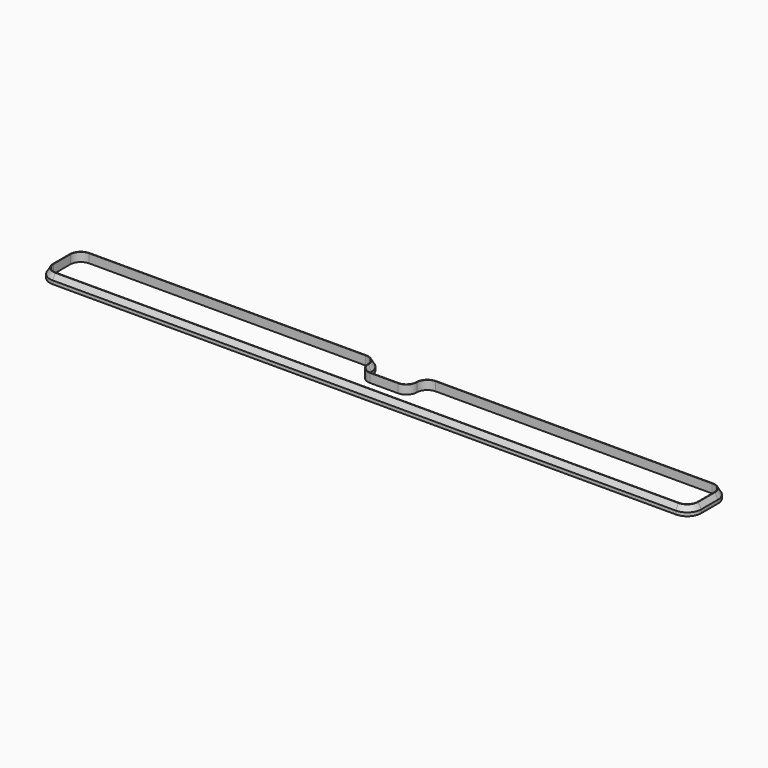
from build123d import *

# Parameters (mm, degrees)
F1_DEPTH = 8.5
F3_DEPTH = 8.501
F5_DEPTH = 8.501
F6_R     = 13.49999
F7_SIZE2 = 5.1961524227
F7_SIZE  = 3


# Not quite as in the source:
# - a fillet or chamfer is up to 0.001 mm smaller than in the source, because OpenCascade refuses the exact size


with BuildPart() as f1:
    # F0 (on Top) → F1 (new body)
    with BuildSketch(Plane.XY):
        with BuildLine():
            Line((-298.5, -23.5), (298.5, -23.5))
            ThreePointArc((298.5, -23.5), (308.045941546, -19.545941546), (312, -10))
            Line((312, -10), (312, 10))
            ThreePointArc((312, 10), (308.045941546, 19.545941546), (298.5, 23.5))
            Line((298.5, 23.5), (-298.5, 23.5))
            ThreePointArc((-298.5, 23.5), (-308.045941546, 19.545941546), (-312, 10))
            Line((-312, 10), (-312, -10))
            ThreePointArc((-312, -10), (-308.045941546, -19.545941546), (-298.5, -23.5))
        make_face()
    extrude(amount=F1_DEPTH)

    # F2 (on face) → F3 (cut, through all)
    with BuildSketch(Plane.XY.offset(8.5)):
        with BuildLine():
            Line((-13.5, 3.5), (13.5, 3.5))
            ThreePointArc((13.5, 3.5), (18.0961940777, 5.4038059223), (20, 10))
            Line((20, 10), (20, 23.5))
            Line((20, 23.5), (-20, 23.5))
            Line((-20, 23.5), (-20, 10))
            ThreePointArc((-20, 10), (-18.0961940777, 5.4038059223), (-13.5, 3.5))
        make_face()
    extrude(amount=-F3_DEPTH, mode=Mode.SUBTRACT)

    # F4 (on face) → F5 (cut, through all)
    with BuildSketch(Plane.XY.offset(8.5)):
        with BuildLine():
            Line((-308.5, 10), (-308.5, -10))
            ThreePointArc((-308.5, -10), (-305.5710678119, -17.0710678119), (-298.5, -20))
            Line((-298.5, -20), (298.5, -20))
            ThreePointArc((298.5, -20), (305.5710678119, -17.0710678119), (308.5, -10))
            Line((308.5, -10), (308.5, 10))
            ThreePointArc((308.5, 10), (305.5710678119, 17.0710678119), (298.5, 20))
            Line((298.5, 20), (33.5, 20))
            ThreePointArc((33.5, 20), (26.4289321881, 17.0710678119), (23.5, 10))
            ThreePointArc((23.5, 10), (20.5710678119, 2.9289321881), (13.5, 0))
            Line((13.5, 0), (-13.5, 0))
            ThreePointArc((-13.5, 0), (-20.5710678119, 2.9289321881), (-23.5, 10))
            ThreePointArc((-23.5, 10), (-26.4289321881, 17.0710678119), (-33.5, 20))
            Line((-33.5, 20), (-298.5, 20))
            ThreePointArc((-298.5, 20), (-305.5710678119, 17.0710678119), (-308.5, 10))
        make_face()
    extrude(amount=-F5_DEPTH, mode=Mode.SUBTRACT)

    # F6 (radius 13.5 in the source; OpenCascade refuses exactly that, so slightly less here)
    f6_edges = [f1.edges().sort_by_distance(p)[0] for p in [
        (-20, 23.5, 4.25),
        (20, 23.5, 4.25),
    ]]
    fillet(f6_edges, radius=F6_R)

    # F7
    f7_edges = [f1.edges().sort_by_distance(p)[0] for p in [
        (165.999995, 23.5, 8.5),
    ]]
    f7_side = f1.faces().sort_by_distance((-165.999995, 22.874232, 8.5))[0]
    chamfer(f7_edges, length=F7_SIZE, length2=F7_SIZE2, reference=f7_side)


solid = f1.part
